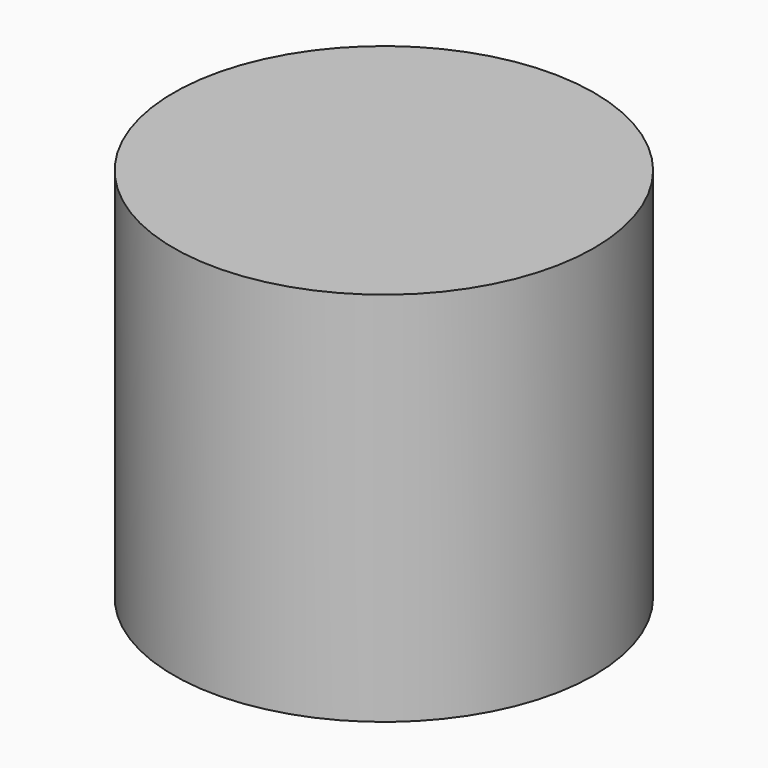
from build123d import *

# Parameters (mm, degrees)
F0_R     = 70.9964788271
F1_DEPTH = 127


# Not quite as in the source:
# - the program builds the solid bodies; features that only make, move or delete a surface that nothing else refers to are left out


with BuildPart() as f1:
    # F0 (on Top) → F1 (new body)
    with BuildSketch(Plane.XY):
        Circle(F0_R)
    extrude(amount=F1_DEPTH)


solid = f1.part
